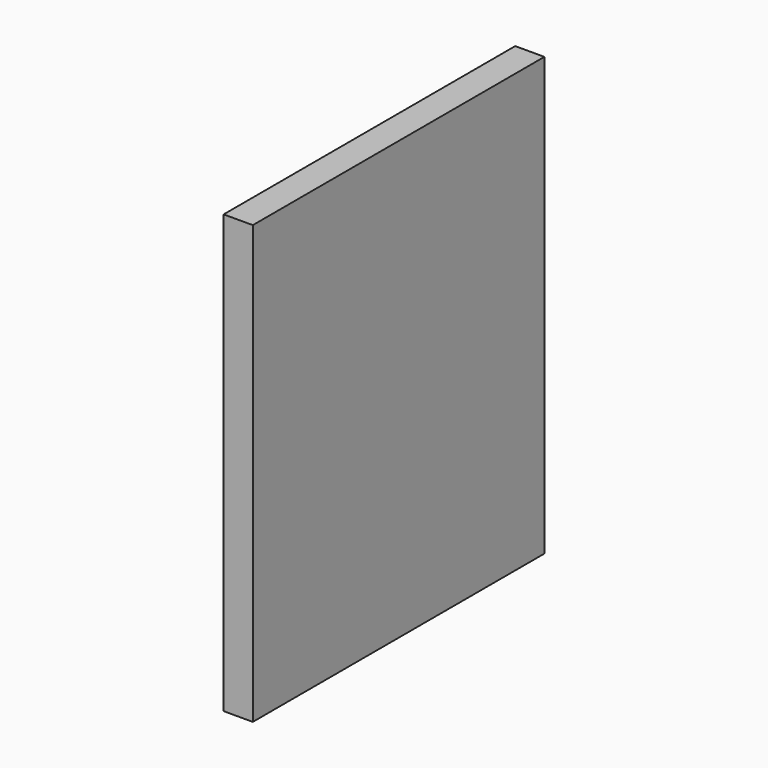
from build123d import *

# Parameters (mm, degrees)
F0_W          = 2500
F0_H          = 3000
F1_DEPTH      = 200
F3_W          = 426.9148111343
F3_H          = 696.6971158981
F6_W          = 348.733663559
F6_H          = 752.1176934242
F7_REACH      = 1496.9403717534
F8_W          = 1770.8705961704
F8_H          = 767.5788402557
F9_DEPTH      = 50
F10_TEXT_SIZE = 327.1314659579
F11_DEPTH     = 50
F12_W         = 375
F12_H         = 500
F12_TEXT_SIZE = 205.8484547964
F13_DEPTH     = 10


# Not quite as in the source:
# - Text() gives the source's letters only with a copy of the font that has no kerning and outlines rounded to 1/6400 em; it was checked with that copy


with BuildPart() as f1:
    # F0 (on Right) → F1 (new body)
    with BuildSketch(Plane.YZ):
        with Locations((1250, 1500)):
            Rectangle(F0_W, F0_H)
    extrude(amount=-F1_DEPTH)

    # F3 (on face) → F4 (join, up to the next surface of F1)
    with BuildSketch(Plane(origin=(-193.9692620786, 0, -34.2020143326), x_dir=(0, 1, 0), z_dir=(0.984807753, 0, 0.1736481777))):
        with Locations((2172.6641058922, 1048.8705039024)):
            Rectangle(F3_W, F3_H)
    extrude(until=Until.NEXT)

    f7_end = Plane(origin=(-200, 1211.2861212798, 1519.7296308955), x_dir=(0, 0, -1), z_dir=(-1, 0, 0))
    # F6 (on face) → F7 (cut, up to a plane its end follows)
    with BuildSketch(Plane(origin=(-144.728874428, 0, -25.5196054492), x_dir=(0, 1, 0), z_dir=(0.984807753, 0, 0.1736481777))):
        with Locations((2175.2992868423, 1106.8154275417)):
            Rectangle(F6_W, F6_H)
    f7_long = extrude(amount=F7_REACH, mode=Mode.PRIVATE)
    add(split(f7_long, bisect_by=f7_end, keep=Keep.TOP, mode=Mode.PRIVATE), mode=Mode.SUBTRACT)

    # F8 (on face) → F9 (join)
    with BuildSketch(Plane(origin=(-200, 0, 0), x_dir=(0, -1, 0), z_dir=(-1, 0, 0))):
        with Locations((-1175.8788079023, 2030.6473970413)):
            Rectangle(F8_W, F8_H)
    extrude(amount=F9_DEPTH)

    # F10 (on face) → F11 (join)
    with BuildSketch(Plane(origin=(-250, 0, 0), x_dir=(0, -1, 0), z_dir=(-1, 0, 0))):
        with Locations((-1592.2209683907, 2152.0953298952)):
            Text('User', F10_TEXT_SIZE, font='Open Sans', font_style=FontStyle.BOLD, text_align=(TextAlign.LEFT, TextAlign.BOTTOM))
        with Locations((-1932.2332358206, 1707.1965361925)):
            Text('Interface', F10_TEXT_SIZE, font='Open Sans', font_style=FontStyle.BOLD, text_align=(TextAlign.LEFT, TextAlign.BOTTOM))
    extrude(amount=F11_DEPTH)

    # F12 (on face) → F13 (join)
    with BuildSketch(Plane(origin=(-200, 0, 0), x_dir=(0, -1, 0), z_dir=(-1, 0, 0))):
        with Locations((-1366.4499078104, 916.3609824601)):
            Rectangle(F12_W, F12_H)
        with Locations((-758.4289989779, 908.0015209586)):
            Rectangle(F12_W, F12_H)
        with Locations((-227.2452495405, 904.4405010611)):
            Rectangle(F12_W, F12_H)
        with Locations((-2452.1600246429, 462.4649410864)):
            Text('Waste    Water Larva Fert', F12_TEXT_SIZE, font='Open Sans', text_align=(TextAlign.LEFT, TextAlign.BOTTOM))
    extrude(amount=F13_DEPTH)


solid = f1.part
